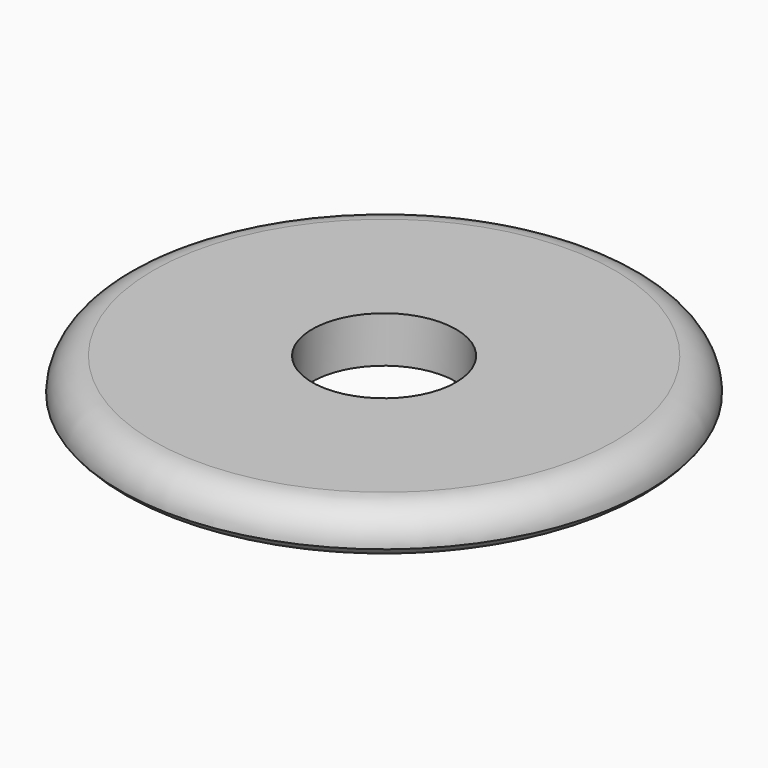
from build123d import *

# Parameters (mm, degrees)
F0_R     = 40
F0_R_2   = 10.9
F1_DEPTH = 7
F2_R     = 5


# Not quite as in the source:
# - a fillet or chamfer that OpenCascade refuses, or shapes differently, is made with other operations: its cross-section is extruded or revolved along the edge and cut away or added


with BuildPart() as f1:
    # F0 (on Top) → F1 (new body)
    with BuildSketch(Plane.XY):
        Circle(F0_R)
        Circle(F0_R_2, mode=Mode.SUBTRACT)
    extrude(amount=F1_DEPTH)

    # F2
    f2_edges = [f1.edges().sort_by_distance(p)[0] for p in [
        (-40, 0, 7),
    ]]
    fillet(f2_edges, radius=F2_R)

    # F3: fillet of radius 5 on 1 edges, made by hand

    # F3_s1 → F3_t2 (revolve, cut)
    with BuildSketch(Plane.XZ):
        with BuildLine():
            ThreePointArc((40, 2), (38.2360679775, 0.527864045), (36, 0))
            Line((36, 0), (40, 0))
            Line((40, 0), (40, 2))
        make_face()
    revolve(axis=Axis((0, 0, 0), (0, 0, 1)), mode=Mode.SUBTRACT)


solid = f1.part
